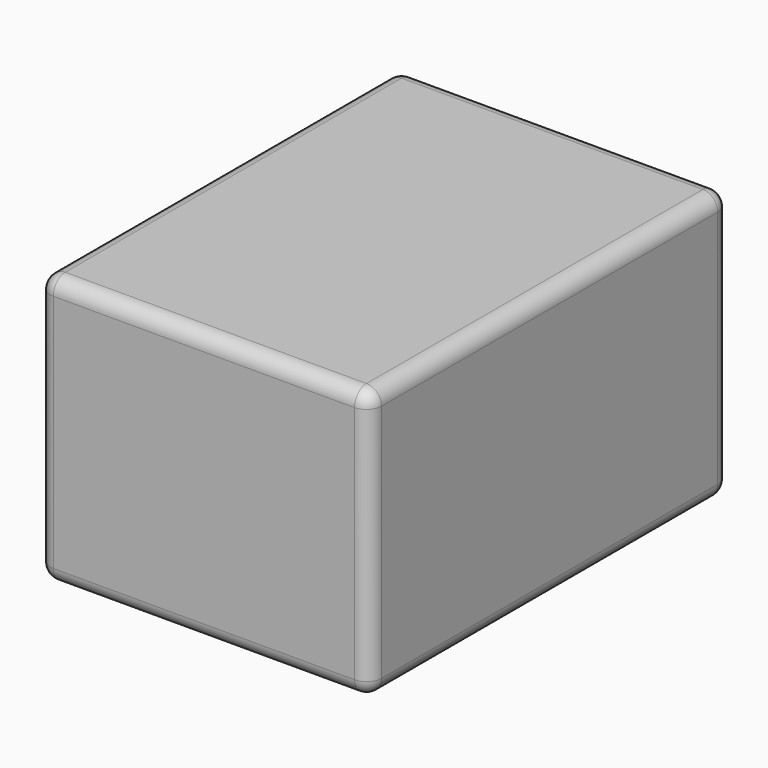
from build123d import *

# Parameters (mm, degrees)
F0_W         = 280.3089916706
F0_H         = 228.1326651573
F1_DEPTH     = 381
F2_R         = 12.7
F3_R         = 12.7
F4_R         = 12.7
F5_T1_DEPTH  = 202.7326651573
F5_T3_DEPTH  = 355.6
F5_T5_DEPTH  = 254.9089916706
F5_S9_W      = 12.7
F5_S9_H      = 12.7
F5_T10_DEPTH = 12.7
F5_S15_W     = 12.7
F5_S15_H     = 12.7
F5_T16_DEPTH = 12.7
F5_T20_ANGLE = 90
F5_T22_ANGLE = 90
F5_T24_ANGLE = 90
F5_T26_ANGLE = 90


# Not quite as in the source:
# - a fillet or chamfer that OpenCascade refuses, or shapes differently, is made with other operations: its cross-section is extruded or revolved along the edge and cut away or added


with BuildPart() as f1:
    # F0 (on Front) → F1 (new body)
    with BuildSketch(Plane.XZ):
        Rectangle(F0_W, F0_H)
    extrude(amount=F1_DEPTH)

    # F2
    f2_edges = [f1.edges().sort_by_distance(p)[0] for p in [
        (0, -381, 114.066333),
    ]]
    fillet(f2_edges, radius=F2_R)

    # F3
    f3_edges = [f1.edges().sort_by_distance(p)[0] for p in [
        (140.154496, -184.15, 114.066333),
        (0, 0, 114.066333),
        (-140.154496, -184.15, 114.066333),
    ]]
    fillet(f3_edges, radius=F3_R)

    # F4
    f4_edges = [f1.edges().sort_by_distance(p)[0] for p in [
        (0, 0, -114.066333),
    ]]
    fillet(f4_edges, radius=F4_R)

    # F5: fillet of radius 12.7 on 1 edges, made by hand

    # F5_s2 → F5_t1 (cut)
    with BuildSketch(Plane.XY.offset(-101.3663325787)):
        with BuildLine():
            ThreePointArc((-127.4544958353, 0), (-136.4347519564, -3.7197438789), (-140.1544958353, -12.7))
            Line((-140.1544958353, -12.7), (-140.1544958353, 0))
            Line((-140.1544958353, 0), (-127.4544958353, 0))
        make_face()
        with BuildLine():
            ThreePointArc((140.1544958353, -12.7), (136.4347519564, -3.7197438789), (127.4544958353, 0))
            Line((127.4544958353, 0), (140.1544958353, 0))
            Line((140.1544958353, 0), (140.1544958353, -12.7))
        make_face()
    extrude(amount=F5_T1_DEPTH, mode=Mode.SUBTRACT)

    # F5_s4 → F5_t3 (cut)
    with BuildSketch(Plane.XZ.offset(12.7)):
        with BuildLine():
            ThreePointArc((-127.4544958353, -114.0663325787), (-136.4347519564, -110.3465886997), (-140.1544958353, -101.3663325787))
            Line((-140.1544958353, -101.3663325787), (-140.1544958353, -114.0663325787))
            Line((-140.1544958353, -114.0663325787), (-127.4544958353, -114.0663325787))
        make_face()
        with BuildLine():
            ThreePointArc((140.1544958353, -101.3663325787), (136.4347519564, -110.3465886997), (127.4544958353, -114.0663325787))
            Line((127.4544958353, -114.0663325787), (140.1544958353, -114.0663325787))
            Line((140.1544958353, -114.0663325787), (140.1544958353, -101.3663325787))
        make_face()
    extrude(amount=F5_T3_DEPTH, mode=Mode.SUBTRACT)

    # F5_s6 → F5_t5 (cut)
    with BuildSketch(Plane.YZ.offset(-127.4544958353)):
        with BuildLine():
            ThreePointArc((-368.3, -114.0663325787), (-377.2802561211, -110.3465886997), (-381, -101.3663325787))
            Line((-381, -101.3663325787), (-381, -114.0663325787))
            Line((-381, -114.0663325787), (-368.3, -114.0663325787))
        make_face()
    extrude(amount=F5_T5_DEPTH, mode=Mode.SUBTRACT)


with BuildPart() as f5_tool8:
    # F5_s9 → F5_t10 (new body)
    with BuildSketch(Plane.XZ.offset(12.7)):
        with Locations((-133.8044958353, 107.7163325787)):
            Rectangle(F5_S9_W, F5_S9_H)
    extrude(amount=-F5_T10_DEPTH)

    # F5_s11 → F5_t12 (revolve, cut)
    with BuildSketch(Plane(origin=(-127.4544958353, -12.7, 101.3663325787), x_dir=(0.7071067812, 0, -0.7071067812), z_dir=(0.7071067812, 0, 0.7071067812))):
        with BuildLine():
            ThreePointArc((0, -12.7), (12.7, 0), (0, 12.7))
            Line((0, 12.7), (0, -12.7))
        make_face()
    revolve(axis=Axis((-127.4544958353, -12.7, 101.3663325787), (0, 1, 0)), mode=Mode.SUBTRACT)


with BuildPart() as f1_1:
    add(f1.part)

    # F5_t7: cut F5_tool8
    add(f5_tool8.part, mode=Mode.SUBTRACT)


with BuildPart() as f5_tool14:
    # F5_s15 → F5_t16 (new body)
    with BuildSketch(Plane.YZ.offset(127.4544958353)):
        with Locations((-6.35, 107.7163325787)):
            Rectangle(F5_S15_W, F5_S15_H)
    extrude(amount=F5_T16_DEPTH)

    # F5_s17 → F5_t18 (revolve, cut)
    with BuildSketch(Plane(origin=(127.4544958353, -12.7, 101.3663325787), x_dir=(0, -0.7071067812, -0.7071067812), z_dir=(0, -0.7071067812, 0.7071067812))):
        with BuildLine():
            ThreePointArc((0, -12.7), (12.7, 0), (0, 12.7))
            Line((0, 12.7), (0, -12.7))
        make_face()
    revolve(axis=Axis((127.4544958353, -12.7, 101.3663325787), (1, 0, 0)), mode=Mode.SUBTRACT)


with BuildPart() as f1_2:
    add(f1_1.part)

    # F5_t13: cut F5_tool14
    add(f5_tool14.part, mode=Mode.SUBTRACT)

    # F5_s19 → F5_t20 (revolve, cut)
    with BuildSketch(Plane.XY.offset(-101.3663325787)):
        with BuildLine():
            ThreePointArc((-127.4544958353, 0), (-136.4347519564, -3.7197438789), (-140.1544958353, -12.7))
            Line((-140.1544958353, -12.7), (-140.1544958353, 0))
            Line((-140.1544958353, 0), (-127.4544958353, 0))
        make_face()
    revolve(axis=Axis((-140.1544958353, -12.7, -101.3663325787), (-1, 0, 0)), revolution_arc=F5_T20_ANGLE, mode=Mode.SUBTRACT)

    # F5_s21 → F5_t22 (revolve, cut)
    with BuildSketch(Plane.YZ.offset(-127.4544958353)):
        with BuildLine():
            ThreePointArc((-368.3, -114.0663325787), (-377.2802561211, -110.3465886997), (-381, -101.3663325787))
            Line((-381, -101.3663325787), (-381, -114.0663325787))
            Line((-381, -114.0663325787), (-368.3, -114.0663325787))
        make_face()
    revolve(axis=Axis((-127.4544958353, -368.3, -114.0663325787), (0, 0, -1)), revolution_arc=F5_T22_ANGLE, mode=Mode.SUBTRACT)

    # F5_s23 → F5_t24 (revolve, cut)
    with BuildSketch(Plane.XZ.offset(368.3)):
        with BuildLine():
            ThreePointArc((127.4544958353, -114.0663325787), (136.4347519564, -110.3465886997), (140.1544958353, -101.3663325787))
            Line((140.1544958353, -101.3663325787), (140.1544958353, -114.0663325787))
            Line((140.1544958353, -114.0663325787), (127.4544958353, -114.0663325787))
        make_face()
    revolve(axis=Axis((127.4544958353, -368.3, -114.0663325787), (0, 0, -1)), revolution_arc=F5_T24_ANGLE, mode=Mode.SUBTRACT)

    # F5_s25 → F5_t26 (revolve, cut)
    with BuildSketch(Plane.XY.offset(-101.3663325787)):
        with BuildLine():
            ThreePointArc((140.1544958353, -12.7), (136.4347519564, -3.7197438789), (127.4544958353, 0))
            Line((127.4544958353, 0), (140.1544958353, 0))
            Line((140.1544958353, 0), (140.1544958353, -12.7))
        make_face()
    revolve(axis=Axis((140.1544958353, -12.7, -101.3663325787), (-1, 0, 0)), revolution_arc=F5_T26_ANGLE, mode=Mode.SUBTRACT)


solid = f1_2.part
